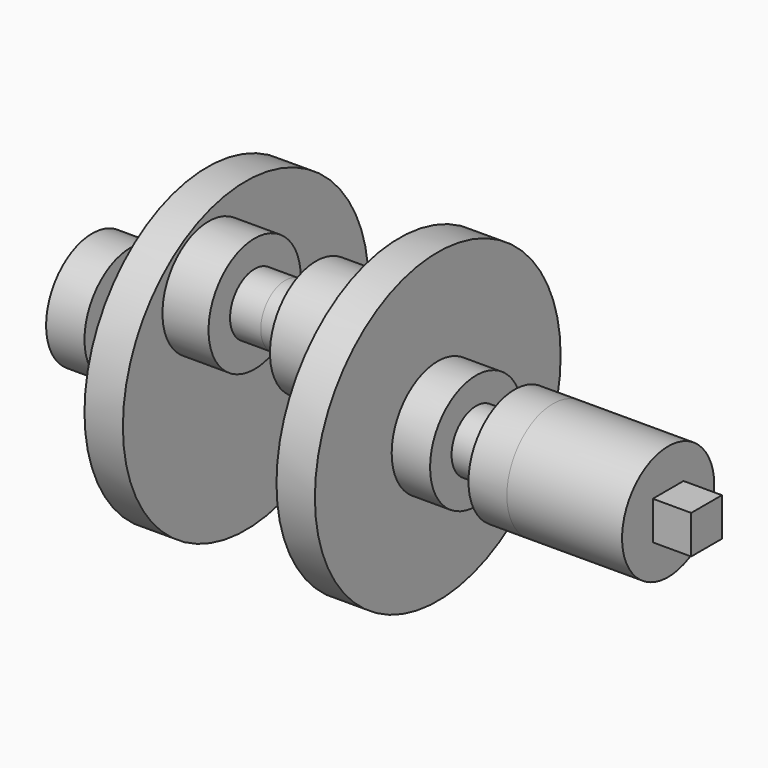
from build123d import *

# Parameters (mm, degrees)
F0_R      = 20
F1_DEPTH  = 5
F3_R      = 7.5
F4_DEPTH  = 5
F5_R      = 4
F6_DEPTH  = 5
F7_R      = 7.5
F7_R_2    = 4
F8_DEPTH  = 5
F2_R      = 7.5
F9_DEPTH  = 6
F10_R     = 4
F11_DEPTH = 4
F13_R     = 7.5
F14_DEPTH = 15
F15_W     = 5
F15_H     = 5
F16_DEPTH = 5


with BuildPart() as f1:
    # F0 (on Right) → F1 (new body)
    with BuildSketch(Plane.YZ):
        with Locations((17.2490278537, 0)):
            Circle(F0_R)
    extrude(amount=F1_DEPTH)

    # F3 (on face) → F4 (join)
    with BuildSketch(Plane(origin=(0, 0, 0), x_dir=(0, -1, 0), z_dir=(-1, 0, 0))):
        with Locations((-17.2490278537, 0)):
            Circle(F3_R)
    extrude(amount=F4_DEPTH)

    # F5 (on face) → F6 (join)
    with BuildSketch(Plane(origin=(-5, 0, 0), x_dir=(0, -1, 0), z_dir=(-1, 0, 0))):
        with Locations((-17.2490278537, 0)):
            Circle(F5_R)
    extrude(amount=F6_DEPTH)

    # F7 (on face) → F8 (join)
    with BuildSketch(Plane(origin=(-10, 0, 0), x_dir=(0, -1, 0), z_dir=(-1, 0, 0))):
        with Locations((-17.2490278537, 0)):
            Circle(F7_R)
        with Locations((-17.2490278537, 0)):
            Circle(F7_R_2, mode=Mode.SUBTRACT)
        with Locations((-17.2490278537, 0)):
            Circle(F7_R_2)
    extrude(amount=F8_DEPTH)

    # F2 (on face) → F9 (join)
    with BuildSketch(Plane.YZ.offset(5)):
        with Locations((11.1903151186, 10.3581851689)):
            Circle(F2_R)
    extrude(amount=F9_DEPTH)

    # F10 (on face) → F11 (join)
    with BuildSketch(Plane.YZ.offset(11)):
        with Locations((11.1903151186, 10.3581851689)):
            Circle(F10_R)
    extrude(amount=F11_DEPTH)

    # F12: F1 across face


with BuildPart() as f1_1:
    add(f1.part)
    add(f1.part.mirror(Plane(origin=(15, 11.1903151186, 10.3581851689), x_dir=(0, 1, 0), z_dir=(1, 0, 0))))

    # F13 (on face) → F14 (join)
    with BuildSketch(Plane.YZ.offset(45)):
        with Locations((17.2490278537, 0)):
            Circle(F13_R)
    extrude(amount=F14_DEPTH)

    # F15 (on face) → F16 (join)
    with BuildSketch(Plane.YZ.offset(60)):
        with Locations((17.2490278537, 0)):
            Rectangle(F15_W, F15_H)
    extrude(amount=F16_DEPTH)


solid = f1_1.part
